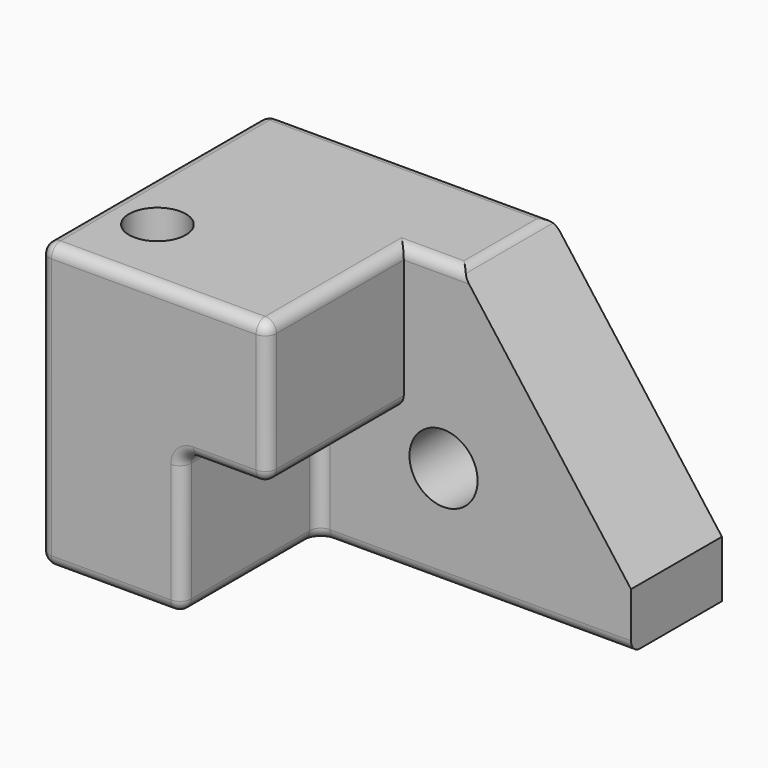
from build123d import *

# Parameters (mm, degrees)
F0_W     = 203.2
F0_H     = 127
F1_DEPTH = 127
F3_DEPTH = 76.2
F4_SIZE2 = 101.6
F4_SIZE  = 76.2
F5_R     = 5.08
F6_R     = 15.24
F7_DEPTH = 50.8
F8_R     = 12.7
F9_DEPTH = 127


with BuildPart() as f1:
    # F0 (on Front) → F1 (new body)
    with BuildSketch(Plane.XZ):
        with Locations((15.3181515634, -8.0336100439)):
            Rectangle(F0_W, F0_H)
    extrude(amount=F1_DEPTH)

    # F2 (on face) → F3 (cut)
    with BuildSketch(Plane.XZ.offset(127)):
        Polygon((-22.7818484366, -8.0336100439), (-22.7818484366, -71.5336100439), (116.9181515634, -71.5336100439), (116.9181515634, 55.4663899561), (15.3181515634, 55.4663899561), (15.3181515634, 37.2199955379), (15.3181515634, -8.0336100439), align=None)
    extrude(amount=-F3_DEPTH, mode=Mode.SUBTRACT)

    # F4
    f4_edges = [f1.edges().sort_by_distance(p)[0] for p in [
        (116.918152, -25.4, 55.46639),
    ]]
    f4_side = f1.faces().sort_by_distance((-6.453277, -52.614286, 55.46639))[0]
    chamfer(f4_edges, length=F4_SIZE, length2=F4_SIZE2, reference=f4_side)

    # F5
    f5_edges = [f1.edges().sort_by_distance(p)[0] for p in [
        (15.318152, -88.9, 55.46639),
        (-35.481848, -127, 55.46639),
        (15.318152, -127, 23.71639),
        (15.318152, -88.9, -8.03361),
        (-22.781848, -88.9, -8.03361),
        (-22.781848, -88.9, -71.53361),
        (-22.781848, -127, -39.78361),
        (-22.781848, -50.8, -39.78361),
        (-3.731848, -127, -8.03361),
        (-54.531848, -127, -71.53361),
        (-86.281848, -127, -8.03361),
        (-86.281848, -63.5, 55.46639),
        (-86.281848, -63.5, -71.53361),
        (-86.281848, 0, -8.03361),
        (-22.781848, 0, 55.46639),
        (40.718152, -25.4, 55.46639),
        (28.018152, -50.8, 55.46639),
        (47.068152, -50.8, -71.53361),
    ]]
    fillet(f5_edges, radius=F5_R)

    # F6 (on face) → F7 (cut, through all)
    with BuildSketch(Plane.XZ.offset(50.8)):
        with Locations((33.0981515634, -25.8136100439)):
            Circle(F6_R)
    extrude(amount=-F7_DEPTH, mode=Mode.SUBTRACT)

    # F8 (on face) → F9 (cut, through all)
    with BuildSketch(Plane.XY.offset(55.4663899561)):
        with Locations((-62.5347197056, -91.1505147815)):
            Circle(F8_R)
    extrude(amount=-F9_DEPTH, mode=Mode.SUBTRACT)


solid = f1.part
